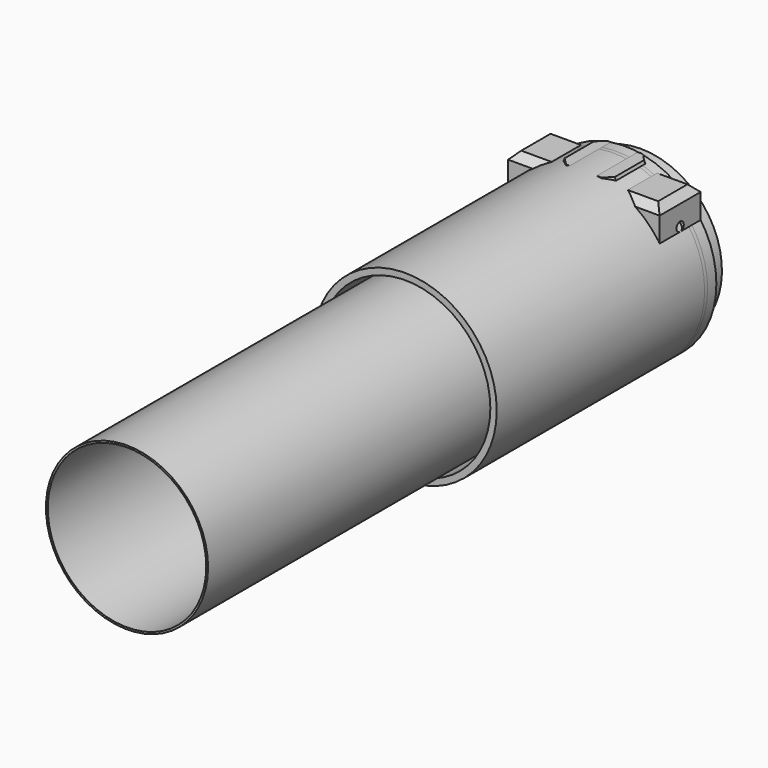
from build123d import *

# Parameters (mm, degrees)
F0_R         = 41.4
F0_R_2       = 31.4
F1_DEPTH     = 65.5
F2_SIZE      = 3
F3_R         = 34
F3_R_2       = 25.4
F4_DEPTH     = 15
F5_R         = 29
F5_R_2       = 25.4
F6_DEPTH     = 120
F7_SIZE2     = 2
F7_SIZE      = 1
F11_DEPTH    = 28
F13_D        = 5
F14_T1_DEPTH = 28
F15_SIZE     = 4
F19_D        = 5
F22_SIZE     = 1
F25_SIZE     = 1
F26_R        = 44.3
F26_R_2      = 43.3
F27_DEPTH    = 340
F28_R        = 50
F28_R_2      = 46.5
F29_DEPTH    = 150
F30_R        = 50
F30_R_2      = 46.5
F31_DEPTH    = 8
F32_SIZE2    = 2.5
F32_SIZE     = 6


# Not quite as in the source:
# - a fillet or chamfer that OpenCascade refuses, or shapes differently, is made with other operations: its cross-section is extruded or revolved along the edge and cut away or added


with BuildPart() as f1:
    # F0 (on Front) → F1 (new body)
    with BuildSketch(Plane.XZ):
        Circle(F0_R)
        Circle(F0_R_2, mode=Mode.SUBTRACT)
    extrude(amount=F1_DEPTH)

    # F2
    f2_edges = [f1.edges().sort_by_distance(p)[0] for p in [
        (-41.4, -65.5, 0),
    ]]
    chamfer(f2_edges, length=F2_SIZE)


with BuildPart() as f4:
    # F3 (on Front) → F4 (new body)
    with BuildSketch(Plane.XZ):
        Circle(F3_R)
        Circle(F3_R_2, mode=Mode.SUBTRACT)
    extrude(amount=F4_DEPTH)

    # F5 (on face) → F6 (join)
    with BuildSketch(Plane.XZ.offset(15)):
        Circle(F5_R)
        Circle(F5_R_2, mode=Mode.SUBTRACT)
    extrude(amount=F6_DEPTH)

    # F7
    f7_edges = [f4.edges().sort_by_distance(p)[0] for p in [
        (-34, 0, 0),
    ]]
    f7_side = f4.faces().sort_by_distance((-34, -7.5, 0))[0]
    chamfer(f7_edges, length=F7_SIZE, length2=F7_SIZE2, reference=f7_side)


with BuildPart() as f9:
    # F8 (on Right) → F9 (revolve)
    with BuildSketch(Plane.YZ):
        Polygon((0, 41.4), (0, 38.4), (10.9333889304, 38.4), (10.9333889304, 44.3), (3.4333889304, 44.3), (1, 41.4), align=None)
    revolve(axis=Axis((0, 5.4666944652, 0), (0, 1, 0)))


with BuildPart() as f11:
    # F10 (on Front) → F11 (new body)
    with BuildSketch(Plane.XZ):
        with BuildLine():
            Line((-41.4, 45.4), (-41.4, 13))
            Line((-41.4, 13), (-39.3059791889, 13))
            ThreePointArc((-39.3059791889, 13), (0, 41.4), (39.3059791889, 13))
            Line((39.3059791889, 13), (41.4, 13))
            Line((41.4, 13), (41.4, 45.4))
            Line((41.4, 45.4), (13.75, 45.4))
            Line((13.75, 45.4), (13.75, 49.4))
            Line((13.75, 49.4), (-13.75, 49.4))
            Line((-13.75, 49.4), (-13.75, 45.4))
            Line((-13.75, 45.4), (-41.4, 45.4))
        make_face()
    extrude(amount=F11_DEPTH)

    # F13 (through all)
    with Locations(Plane.XY.offset(49.4)):
        with Locations((0, -22.5)):
            Hole(F13_D / 2)

    # F14: fillet of radius 5 on 2 edges, made by hand

    # F14_s2 → F14_t1 (join)
    with BuildSketch(Plane.XZ):
        with BuildLine():
            ThreePointArc((18.6489794856, 45.4), (15.4867018254, 46.5270166538), (13.75, 49.4))
            Line((13.75, 49.4), (13.75, 45.4))
            Line((13.75, 45.4), (18.6489794856, 45.4))
        make_face()
        with BuildLine():
            ThreePointArc((-18.6489794856, 45.4), (-15.4867018254, 46.5270166538), (-13.75, 49.4))
            Line((-13.75, 49.4), (-13.75, 45.4))
            Line((-13.75, 45.4), (-18.6489794856, 45.4))
        make_face()
    extrude(amount=F14_T1_DEPTH)

    # F15
    f15_edges = [f11.edges().sort_by_distance(p)[0] for p in [
        (-30.02449, -28, 45.4),
        (-41.4, -14, 45.4),
        (-30.02449, 0, 45.4),
        (30.02449, 0, 45.4),
        (41.4, -14, 45.4),
        (30.02449, -28, 45.4),
        (15.486702, -28, 46.527017),
        (-15.486702, -28, 46.527017),
    ]]
    chamfer(f15_edges, length=F15_SIZE)

    # F19 (through all)
    with Locations(Plane(origin=(-41.4, 0, 0), x_dir=(0, -1, 0), z_dir=(-1, 0, 0))):
        with Locations((14, 30.4)):
            Hole(F19_D / 2)


with BuildPart() as f17:
    # F16 (on Front) → F17 (revolve)
    with BuildSketch(Plane.XZ):
        Polygon((17.8218007376, 12), (0, 12), (0, 0), (27, 0), (27, 14), (19.5, 14), align=None)
    revolve(axis=Axis((13.5, 0, 0), (-1, 0, 0)))


with BuildPart() as f21:
    # F20 (on Front) → F21 (revolve)
    with BuildSketch(Plane.XZ):
        Polygon((0, 15), (0, 22.5), (-18, 22.5), (-18, 19.5), (-14, 19.5), (-14, 12.75), (-7.5, 12.75), (-7.5, 4.75), (-1.5, 4.75), (-1.5, 15), align=None)
    revolve(axis=Axis((-9, 0, 0), (-1, 0, 0)))

    # F22
    f22_edges = [f21.edges().sort_by_distance(p)[0] for p in [
        (0, 0, -22.5),
        (-18, 0, -22.5),
    ]]
    chamfer(f22_edges, length=F22_SIZE)


with BuildPart() as f24:
    # F23 (on Front) → F24 (revolve)
    with BuildSketch(Plane.XZ):
        Polygon((0, 12), (0, 4.75), (24, 4.75), (24, 0), (27, 0), (27, 22.5), (9, 22.5), (9, 19.4999976456), (24, 19.4999976456), (24, 12), align=None)
    revolve(axis=Axis((25.5, 0, 0), (-1, 0, 0)))

    # F25
    f25_edges = [f24.edges().sort_by_distance(p)[0] for p in [
        (27, 0, -22.5),
        (9, 0, -22.5),
    ]]
    chamfer(f25_edges, length=F25_SIZE)


with BuildPart() as f27:
    # F26 (on Front) → F27 (new body)
    with BuildSketch(Plane.XZ):
        Circle(F26_R)
        Circle(F26_R_2, mode=Mode.SUBTRACT)
    extrude(amount=F27_DEPTH)


with BuildPart() as f29:
    # F28 (on Front) → F29 (new body)
    with BuildSketch(Plane.XZ):
        Circle(F28_R)
        Circle(F28_R_2, mode=Mode.SUBTRACT)
    extrude(amount=F29_DEPTH)


with BuildPart() as f31:
    # F30 (on Front) → F31 (new body)
    with BuildSketch(Plane.XZ):
        Circle(F30_R)
        Circle(F30_R_2, mode=Mode.SUBTRACT)
    extrude(amount=F31_DEPTH)

    # F32
    f32_edges = [f31.edges().sort_by_distance(p)[0] for p in [
        (-50, 0, 0),
    ]]
    f32_side = f31.faces().sort_by_distance((-50, -4, 0))[0]
    chamfer(f32_edges, length=F32_SIZE, length2=F32_SIZE2, reference=f32_side)


solid = Compound([f1.part, f4.part, f9.part, f11.part, f17.part, f21.part, f24.part, f27.part, f29.part, f31.part])
